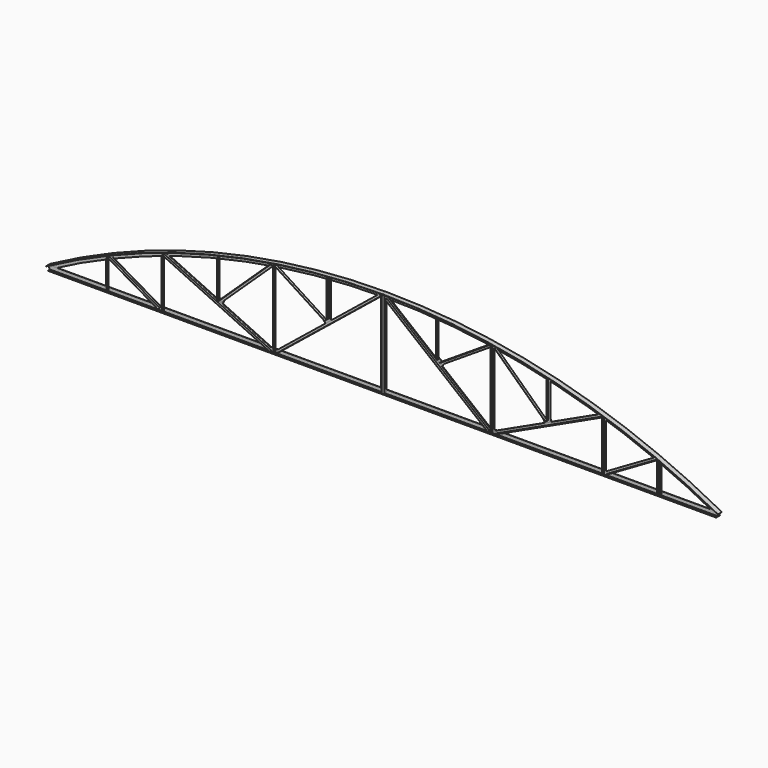
from build123d import *

# Parameters (mm, degrees)
F2_DEPTH  = 18288
F8_DEPTH  = 838.2
F11_DEPTH = 1574.8
F14_DEPTH = 1386.84
F19_DEPTH = 3225.8
F24_DEPTH = 1016
F28_DEPTH = 1917.7
F29_W     = 203.2
F29_H     = 6.35
F30_DEPTH = 76.962
F33_DEPTH = 2120.9
F35_DEPTH = 2379.98
F39_DEPTH = 3614.42
F43_DEPTH = 1021.08
F47_DEPTH = 1617.98
F48_W     = 215.9
F48_H     = 6.35
F49_DEPTH = 91.44


with BuildPart() as f2:
    # F1 (on Right) → F2 (new body, through all)
    with BuildSketch(Plane.YZ):
        Polygon((-68.2625, 3.175), (-68.2625, -3.175), (68.2625, -3.175), (68.2625, 3.175), (3.175, 3.175), (3.175, 104.775), (-3.175, 104.775), (-3.175, 3.175), align=None)
    extrude(amount=F2_DEPTH)

    # F7 (on line) → F8 (join)
    with BuildSketch(Plane.XY):
        Polygon((1606.55, -66.675), (1612.9, -66.675), (1612.9, -3.175), (1549.4, -3.175), (1549.4, -9.525), (1606.55, -9.525), align=None)
    extrude(amount=F8_DEPTH)

    # F34 (on face) → F35 (join)
    with BuildSketch(Plane.XY.offset(3.175)):
        Polygon((9131.7032778758, -66.675), (9131.7032778758, -3.175), (9068.2032778758, -3.175), (9068.2032778758, -9.525), (9125.3532778758, -9.525), (9125.3532778758, -66.675), align=None)
    extrude(amount=F35_DEPTH)


with BuildPart() as f5:
    # F5: sweep along a path in F0
    with BuildLine(Plane.XZ) as f5_path:
        ThreePointArc((18288, 0), (9144, 2305.05), (0, 0))
    # F4 (on line) → F5 (sweep)
    with BuildSketch(Plane(origin=(0, 0, 0), x_dir=(0, -1, 0), z_dir=(-0.8805016303, 0, -0.4740431193))):
        Polygon((-3.175, 3.2512948513), (3.175, 3.2512948513), (3.175, 98.5012948513), (68.2625, 98.5012948513), (68.2625, 104.8512948513), (-68.2625, 104.8512948513), (-68.2625, 98.5012948513), (-3.175, 98.5012948513), align=None)
    sweep(path=f5_path.line)


with BuildPart() as f11:
    # F10 (on line) → F11 (new body)
    with BuildSketch(Plane(origin=(2319.6376904191, 0, -1338.8967700774), x_dir=(0, -1, 0), z_dir=(-0.8660814465, 0, 0.4999029185))):
        Polygon((3.175, 1609.4247804352), (3.175, 1545.9247804352), (66.675, 1545.9247804352), (66.675, 1552.2747804352), (9.525, 1552.2747804352), (9.525, 1609.4247804352), align=None)
    extrude(amount=F11_DEPTH)


with BuildPart() as f14:
    # F13 (on line) → F14 (new body)
    with BuildSketch(Plane.XY):
        Polygon((3118.2980941772, -66.675), (3124.6480941772, -66.675), (3124.6480941772, -9.525), (3124.6480941772, -3.175), (3118.2980941772, -3.175), (3061.1480941772, -3.175), (3061.1480941772, -9.525), (3118.2980941772, -9.525), align=None)
    extrude(amount=F14_DEPTH)


with BuildPart() as f11_1:
    # F15: moved
    add(f11.part.moved(Location((-82.4942577827, 0, 47.6157529908))))


with BuildPart() as f19:
    # F18 (on offset) → F19 (new body)
    with BuildSketch(Plane(origin=(4980.3930912222, 0, -2317.7527969135), x_dir=(0, -1, 0), z_dir=(-0.9066312313, 0, 0.4219239392))):
        Polygon((-66.675, 2580.0859846597), (-3.175, 2580.0859846597), (-3.175, 2643.5859846597), (-9.525, 2643.5859846597), (-9.525, 2586.4359846597), (-66.675, 2586.4359846597), align=None)
    extrude(amount=F19_DEPTH)


with BuildPart() as f19b:
    # F18 (on offset) → F19, piece 2 (new body)
    with BuildSketch(Plane(origin=(4980.3930912222, 0, -2317.7527969135), x_dir=(0, -1, 0), z_dir=(-0.9066312313, 0, 0.4219239392))):
        Polygon((9.525, 2643.5859846597), (3.175, 2643.5859846597), (3.175, 2580.0859846597), (66.675, 2580.0859846597), (66.675, 2586.4359846597), (9.525, 2586.4359846597), align=None)
    extrude(amount=F19_DEPTH)


with BuildPart() as f24:
    # F23 (on offset) → F24 (new body)
    with BuildSketch(Plane.XY.offset(808.1843522508)):
        Polygon((4644.5621094631, -73.025), (4644.5621094631, -9.525), (4581.0621094631, -9.525), (4581.0621094631, -15.875), (4638.2121094631, -15.875), (4638.2121094631, -73.025), align=None)
    extrude(amount=F24_DEPTH)


with BuildPart() as f28:
    # F27 (on offset) → F28 (new body)
    with BuildSketch(Plane(origin=(2859.4838949755, 0, 2704.835345997), x_dir=(0, 1, 0), z_dir=(0.7264787985, 0, 0.687188879))):
        Polygon((-15.3970178679, -2695.1189300565), (-9.0470178679, -2695.1189300565), (-9.0470178679, -2631.6189300565), (-72.5470178679, -2631.6189300565), (-72.5470178679, -2637.9689300565), (-15.3970178679, -2637.9689300565), align=None)
    extrude(amount=F28_DEPTH)


with BuildPart() as f30:
    # F29 (on face) → F30 (new body)
    with BuildSketch(Plane(origin=(1115.3922123716, 0, 2396.7576162119), x_dir=(0.9066312313, 0, -0.4219239392), z_dir=(0.4219239392, 0, 0.9066312313))):
        with Locations((3891.4359298706, -6.35)):
            Rectangle(F29_W, F29_H)
    extrude(amount=F30_DEPTH)


with BuildPart() as f33:
    # F32 (on offset) → F33 (new body)
    with BuildSketch(Plane.XY.offset(3.175)):
        Polygon((6178.55, -3.175), (6115.05, -3.175), (6115.05, -9.525), (6172.2, -9.525), (6172.2, -66.675), (6178.55, -66.675), (6178.55, -9.525), align=None)
    extrude(amount=F33_DEPTH)


with BuildPart() as f39:
    # F38 (on offset) → F39 (new body)
    with BuildSketch(Plane(origin=(3800.6710193181, 0, 3070.690814839), x_dir=(0, 1, 0), z_dir=(0.7778493281, 0, 0.6284508117))):
        Polygon((-4.0887994692, -3906.5081362077), (-4.0887994692, -3843.0081362077), (-10.4387994692, -3843.0081362077), (-10.4387994692, -3900.1581362077), (-67.5887994692, -3900.1581362077), (-67.5887994692, -3906.5081362077), align=None)
    extrude(amount=F39_DEPTH)


with BuildPart() as f39b:
    # F38 (on offset) → F39, piece 2 (new body)
    with BuildSketch(Plane(origin=(3800.6710193181, 0, 3070.690814839), x_dir=(0, 1, 0), z_dir=(0.7778493281, 0, 0.6284508117))):
        Polygon((10.4387994692, -3843.0081362077), (4.0887994692, -3843.0081362077), (4.0887994692, -3906.5081362077), (67.5887994692, -3906.5081362077), (67.5887994692, -3900.1581362077), (10.4387994692, -3900.1581362077), align=None)
    extrude(amount=F39_DEPTH)


with BuildPart() as f43:
    # F42 (on face) → F43 (new body)
    with BuildSketch(Plane.XY.offset(1310.005)):
        Polygon((7638.4372711182, -12.7), (7638.4372711182, -76.2), (7644.7872711182, -76.2), (7644.7872711182, -19.05), (7701.9372711182, -19.05), (7701.9372711182, -12.7), align=None)
    extrude(amount=F43_DEPTH)


with BuildPart() as f47:
    # F46 (on face) → F47 (new body)
    with BuildSketch(Plane(origin=(4785.974791077, 0, -3077.3230314053), x_dir=(0, 1, 0), z_dir=(0.841128511, 0, -0.5408353057))):
        Polygon((-12.6969806187, 5096.0150404202), (-12.6969806187, 5159.5150404202), (-76.2030244117, 5159.5150404202), (-76.2030244117, 5153.1650404202), (-19.0469806187, 5153.1650404202), (-19.0469806187, 5096.1535319751), align=None)
    extrude(amount=-F47_DEPTH)


with BuildPart() as f49:
    # F48 (on face) → F49 (new body)
    with BuildSketch(Plane(origin=(2415.1415826459, 0, -2989.2812966888), x_dir=(0.7778493281, 0, 0.6284508117), z_dir=(-0.6284508117, 0, 0.7778493281))):
        with Locations((6709.1639320374, -7.2637994692)):
            Rectangle(F48_W, F48_H)
    extrude(amount=F49_DEPTH)


with BuildPart() as f51_1:
    # F51: instance of F39
    add(f39.part.mirror(Plane(origin=(9144.4032778758, -34.925, 1193.165), x_dir=(0, 1, 0), z_dir=(1, 0, 0))))


with BuildPart() as f51_2:
    # F51: instance of F43
    add(f43.part.mirror(Plane(origin=(9144.4032778758, -34.925, 1193.165), x_dir=(0, 1, 0), z_dir=(1, 0, 0))))


with BuildPart() as f51_3:
    # F51: instance of F49
    add(f49.part.mirror(Plane(origin=(9144.4032778758, -34.925, 1193.165), x_dir=(0, 1, 0), z_dir=(1, 0, 0))))


with BuildPart() as f51_4:
    # F51: instance of F5
    add(f5.part.mirror(Plane(origin=(9144.4032778758, -34.925, 1193.165), x_dir=(0, 1, 0), z_dir=(1, 0, 0))))


with BuildPart() as f51_5:
    # F51: instance of F33
    add(f33.part.mirror(Plane(origin=(9144.4032778758, -34.925, 1193.165), x_dir=(0, 1, 0), z_dir=(1, 0, 0))))


with BuildPart() as f51_6:
    # F51: instance of F28
    add(f28.part.mirror(Plane(origin=(9144.4032778758, -34.925, 1193.165), x_dir=(0, 1, 0), z_dir=(1, 0, 0))))


with BuildPart() as f51_7:
    # F51: instance of F19
    add(f19.part.mirror(Plane(origin=(9144.4032778758, -34.925, 1193.165), x_dir=(0, 1, 0), z_dir=(1, 0, 0))))


with BuildPart() as f51_8:
    # F51: instance of F19b
    add(f19b.part.mirror(Plane(origin=(9144.4032778758, -34.925, 1193.165), x_dir=(0, 1, 0), z_dir=(1, 0, 0))))


with BuildPart() as f51_9:
    # F51: instance of F24
    add(f24.part.mirror(Plane(origin=(9144.4032778758, -34.925, 1193.165), x_dir=(0, 1, 0), z_dir=(1, 0, 0))))


with BuildPart() as f51_10:
    # F51: instance of F14
    add(f14.part.mirror(Plane(origin=(9144.4032778758, -34.925, 1193.165), x_dir=(0, 1, 0), z_dir=(1, 0, 0))))


with BuildPart() as f51_11:
    # F51: instance of F11
    add(f11_1.part.mirror(Plane(origin=(9144.4032778758, -34.925, 1193.165), x_dir=(0, 1, 0), z_dir=(1, 0, 0))))


with BuildPart() as f51_12:
    # F51: instance of F2
    add(f2.part.mirror(Plane(origin=(9144.4032778758, -34.925, 1193.165), x_dir=(0, 1, 0), z_dir=(1, 0, 0))))


with BuildPart() as f51_13:
    # F51: instance of F39b
    add(f39b.part.mirror(Plane(origin=(9144.4032778758, -34.925, 1193.165), x_dir=(0, 1, 0), z_dir=(1, 0, 0))))


with BuildPart() as f51_14:
    # F51: instance of F30
    add(f30.part.mirror(Plane(origin=(9144.4032778758, -34.925, 1193.165), x_dir=(0, 1, 0), z_dir=(1, 0, 0))))


with BuildPart() as f51_15:
    # F51: instance of F47
    add(f47.part.mirror(Plane(origin=(9144.4032778758, -34.925, 1193.165), x_dir=(0, 1, 0), z_dir=(1, 0, 0))))


solid = Compound([f2.part, f5.part, f14.part, f11_1.part, f19.part, f19b.part, f24.part, f28.part, f30.part, f33.part, f39.part, f39b.part, f43.part, f47.part, f49.part, f51_1.part, f51_2.part, f51_3.part, f51_4.part, f51_5.part, f51_6.part, f51_7.part, f51_8.part, f51_9.part, f51_10.part, f51_11.part, f51_12.part, f51_13.part, f51_14.part, f51_15.part])
